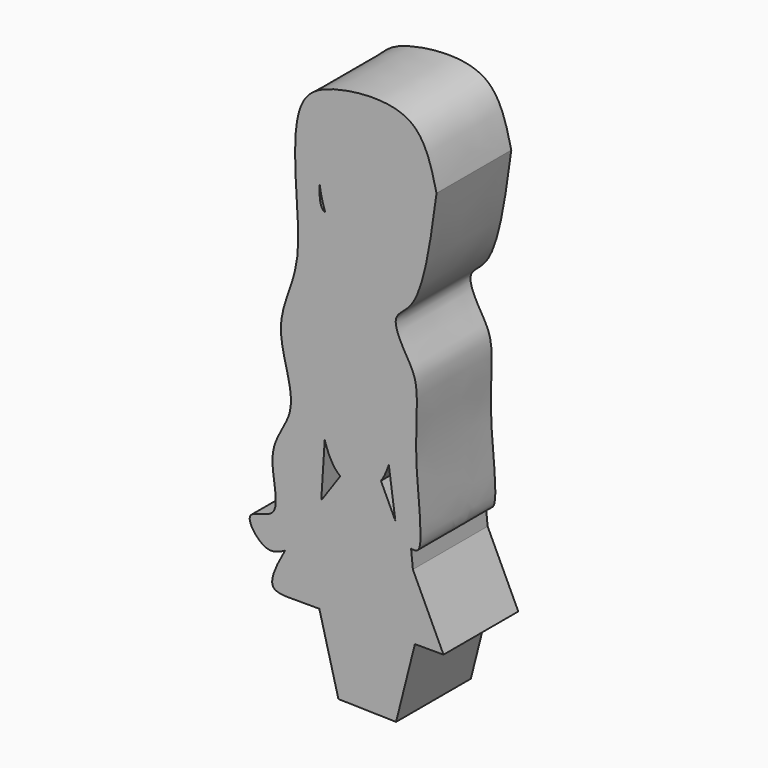
from build123d import *

# Parameters (mm, degrees)
F1_DEPTH = 25.4


with BuildPart() as f1:
    # F0 (on Front) → F1 (new body)
    with BuildSketch(Plane.XZ):
        with BuildLine():
            add(Edge.make_bspline(
                [(-13.2597442659, 48.0586274406), (-13.5977464023, 50.6112678955), (-13.8470723957, 57.8086655511), (-13.1131117441, 63.740427035), (-9.6694547683, 65.7902136445)],
                knots=[0.8065998572, 0.8065998572, 0.8065998572, 0.8065998572, 0.8751143357, 1, 1, 1, 1], degree=3))
            add(Edge.make_bspline(
                [(-9.6694547683, 65.7902136445), (-5.0770227001, 68.5237918796), (8.754968388, 67.9170672824), (13.1442032737, 62.5296557289), (13.9137207846, 60.7951997848)],
                knots=[0, 0, 0, 0, 0.1665464748, 0.23330744, 0.23330744, 0.23330744, 0.23330744], degree=3))
            add(Edge.make_bspline(
                [(13.9137207846, 60.7951997848), (14.5365060561, 59.3914713436), (15.6047629812, 54.0176064848), (14.0449258965, 45.1178162392), (7.561997369, 35.3712418653), (4.3727098317, 32.8274617106)],
                knots=[0.23330744, 0.23330744, 0.23330744, 0.23330744, 0.2873383688, 0.4230765743, 0.5331132448, 0.5331132448, 0.5331132448, 0.5331132448], degree=3))
            add(Edge.make_bspline(
                [(4.3727098317, 32.8274617106), (3.6723806459, 29.8240940225), (2.316637011, 24.0404033145), (4.425251651, 16.2436942218), (6.4598966618, 12.9076730343), (7.3942886665, 11.3758295774)],
                knots=[0, 0, 0, 0, 0.3683955853, 0.7100495981, 1, 1, 1, 1], degree=3))
            add(Edge.make_bspline(
                [(7.3942886665, 11.3758295774), (8.8184184197, -2.9290787173), (10.2432882502, -17.2336376752), (11.667567898, -31.5384752155)],
                knots=[0, 0, 0, 0, 43.1265648658, 43.1265648658, 43.1265648658, 43.1265648658], degree=3))
            add(Edge.make_bspline(
                [(18.5805205256, 55.7415634394), (16.9604621778, 43.7962208668), (14.5923827816, 26.3354173288), (5.783112798, 23.025573274), (9.9611159632, 14.6191299816), (14.2829401574, 8.3648794745), (11.7982647785, -8.4718891545), (15.6711855516, -32.1567528805), (12.4305942317, -31.6563107137), (11.667567898, -31.5384752155)],
                knots=[0, 0, 0, 0, 0.2296881978, 0.3357415022, 0.4503590021, 0.5643656145, 0.7444344835, 0.9398265709, 1, 1, 1, 1], degree=3))
            add(Edge.make_bspline(
                [(18.5805205256, 55.7415634394), (17.1329290258, 61.7846025086), (14.1281204981, 74.3283175814), (-8.5896728026, 72.8654786115), (-20.7194357662, 66.8136292861), (-19.5948869652, 43.7186228989), (-18.5533462423, 29.7113103857), (-20.7946125304, 20.6272816454), (-25.134054069, 10.2812154641), (-21.264747451, -1.7794824434), (-20.2945141104, -11.0677644833), (-28.6889299444, -20.5489013554), (-22.080213584, -37.1533798953), (-35.2491774446, -36.1367283315), (-28.1127555437, -45.9231665153), (-24.3435984622, -44.0537302743), (-22.6038616138, -43.1667872706)],
                knots=[0, 0, 0, 0, 0.085428964, 0.1772788288, 0.2494957552, 0.3459393214, 0.4258178937, 0.4882638252, 0.5568299207, 0.6301735859, 0.6919027853, 0.7637951512, 0.8404855359, 0.8945923927, 0.950900518, 1, 1, 1, 1], degree=3))
            add(Edge.make_bspline(
                [(-12.7485493713, -27.9239041306), (-16.6095460872, -33.5399624759), (-20.1444244224, -38.8530041581), (-22.6038616138, -43.1667872706)],
                knots=[0.1336483622, 0.1336483622, 0.1336483622, 0.1336483622, 0.4407324334, 0.4407324334, 0.4407324334, 0.4407324334], degree=3))
            add(Edge.make_bspline(
                [(-11.8084209481, -13.1750907084), (-12.1196551239, -18.0980314336), (-12.4373151954, -23.0009634054), (-12.7485493713, -27.9239041306)],
                knots=[0, 0, 0, 0, 14.7787461854, 14.7787461854, 14.7787461854, 14.7787461854], degree=3))
            add(Edge.make_bspline(
                [(-11.8084209481, -13.1750907084), (-13.8312312099, -6.5254381988), (-14.4995019899, 3.1835847003), (-15.1677727699, 12.8926075995)],
                knots=[0.7333685705, 0.7333685705, 0.7333685705, 0.7333685705, 1, 1, 1, 1], degree=3))
            add(Edge.make_bspline(
                [(-6.6413877679, 33.3635374314), (-6.2702296071, 30.7940506233), (-5.4996297901, 25.4655688344), (-8.9210699083, 16.2139387081), (-13.1930747657, 13.9425430583), (-15.1677727699, 12.8926075995)],
                knots=[0, 0, 0, 0, 0.3336593067, 0.6920012702, 1, 1, 1, 1], degree=3))
            add(Edge.make_bspline(
                [(-6.6413877679, 33.3635374314), (-8.1182076926, 34.7468870359), (-10.0297540913, 37.3896335016), (-11.3071284072, 40.3375022756), (-11.6578137626, 41.2990598225)],
                knots=[0.6602569137, 0.6602569137, 0.6602569137, 0.6602569137, 0.7180952928, 0.7451794293, 0.7451794293, 0.7451794293, 0.7451794293], degree=3))
            add(Edge.make_bspline(
                [(-11.6578137761, 41.2990598059), (-13.2743628001, 41.8800629418), (-13.2500921799, 44.9736955763), (-13.2597442659, 48.0586274406)],
                knots=[0.6826892363, 0.6826892363, 0.6826892363, 0.6826892363, 1, 1, 1, 1], degree=3))
        make_face()
        with BuildLine():
            add(Edge.make_bspline(
                [(-9.6694547683, 65.7902136445), (-5.0770227001, 68.5237918796), (8.754968388, 67.9170672824), (13.1442032737, 62.5296557289), (13.9137207846, 60.7951997848)],
                knots=[0, 0, 0, 0, 0.1665464748, 0.23330744, 0.23330744, 0.23330744, 0.23330744], degree=3))
            add(Edge.make_bspline(
                [(-13.2597442659, 48.0586274406), (-13.5977464023, 50.6112678955), (-13.8470723957, 57.8086655511), (-13.1131117441, 63.740427035), (-9.6694547683, 65.7902136445)],
                knots=[0.8065998572, 0.8065998572, 0.8065998572, 0.8065998572, 0.8751143357, 1, 1, 1, 1], degree=3))
            add(Edge.make_bspline(
                [(-11.6578137626, 41.2990598225), (-12.4530853654, 43.4796453527), (-12.9567391737, 45.7702896672), (-13.2597442659, 48.0586274406)],
                knots=[0.7451794293, 0.7451794293, 0.7451794293, 0.7451794293, 0.8065998572, 0.8065998572, 0.8065998572, 0.8065998572], degree=3))
            add(Edge.make_bspline(
                [(13.9137207846, 60.7951997848), (2.8933144958, 50.429697228), (-8.1798333223, 40.0490405239), (-11.6578137535, 41.2990597978)],
                knots=[0, 0, 0, 0, 0.6826892348, 0.6826892348, 0.6826892348, 0.6826892348], degree=3))
        make_face()
        with BuildLine():
            add(Edge.make_bspline(
                [(13.9137207846, 60.7951997848), (14.5365060561, 59.3914713436), (15.6047629812, 54.0176064848), (14.0449258965, 45.1178162392), (7.561997369, 35.3712418653), (4.3727098317, 32.8274617106)],
                knots=[0.23330744, 0.23330744, 0.23330744, 0.23330744, 0.2873383688, 0.4230765743, 0.5331132448, 0.5331132448, 0.5331132448, 0.5331132448], degree=3))
            add(Edge.make_bspline(
                [(13.9137207846, 60.7951997848), (2.8933144958, 50.429697228), (-8.1798333223, 40.0490405239), (-11.6578137535, 41.2990597978)],
                knots=[0, 0, 0, 0, 0.6826892348, 0.6826892348, 0.6826892348, 0.6826892348], degree=3))
            add(Edge.make_bspline(
                [(-6.6413877679, 33.3635374314), (-8.1182076926, 34.7468870359), (-10.0297540913, 37.3896335016), (-11.3071284072, 40.3375022756), (-11.6578137626, 41.2990598225)],
                knots=[0.6602569137, 0.6602569137, 0.6602569137, 0.6602569137, 0.7180952928, 0.7451794293, 0.7451794293, 0.7451794293, 0.7451794293], degree=3))
            add(Edge.make_bspline(
                [(4.3727098317, 32.8274617106), (2.9498352275, 31.6925749566), (-0.8831222645, 29.691479536), (-4.6484495647, 31.4967355087), (-6.6413877679, 33.3635374314)],
                knots=[0.5331132448, 0.5331132448, 0.5331132448, 0.5331132448, 0.5822052073, 0.6602569137, 0.6602569137, 0.6602569137, 0.6602569137], degree=3))
        make_face()
        with BuildLine():
            add(Edge.make_bspline(
                [(4.3727098317, 32.8274617106), (3.6723806459, 29.8240940225), (2.316637011, 24.0404033145), (4.425251651, 16.2436942218), (6.4598966618, 12.9076730343), (7.3942886665, 11.3758295774)],
                knots=[0, 0, 0, 0, 0.3683955853, 0.7100495981, 1, 1, 1, 1], degree=3))
            add(Edge.make_bspline(
                [(4.3727098317, 32.8274617106), (2.9498352275, 31.6925749566), (-0.8831222645, 29.691479536), (-4.6484495647, 31.4967355087), (-6.6413877679, 33.3635374314)],
                knots=[0.5331132448, 0.5331132448, 0.5331132448, 0.5331132448, 0.5822052073, 0.6602569137, 0.6602569137, 0.6602569137, 0.6602569137], degree=3))
            add(Edge.make_bspline(
                [(-6.6413877679, 33.3635374314), (-6.2702296071, 30.7940506233), (-5.4996297901, 25.4655688344), (-8.9210699083, 16.2139387081), (-13.1930747657, 13.9425430583), (-15.1677727699, 12.8926075995)],
                knots=[0, 0, 0, 0, 0.3336593067, 0.6920012702, 1, 1, 1, 1], degree=3))
            add(Edge.make_bspline(
                [(-15.1677727699, 12.8926075995), (-11.2202851493, 11.2914109173), (-3.5354144526, 8.17424105), (3.8180690975, 10.3282637453), (7.3942886665, 11.3758295774)],
                knots=[0, 0, 0, 0, 0.5136700117, 1, 1, 1, 1], degree=3))
        make_face()
        with BuildLine():
            add(Edge.make_bspline(
                [(7.3942886665, 11.3758295774), (7.4809183559, 2.1480170491), (7.5675480452, -7.0797954793), (5.6052811607, -13.4339725009)],
                knots=[0, 0, 0, 0, 0.2824189835, 0.2824189835, 0.2824189835, 0.2824189835], degree=3))
            add(Edge.make_bspline(
                [(-15.1677727699, 12.8926075995), (-11.2202851493, 11.2914109173), (-3.5354144526, 8.17424105), (3.8180690975, 10.3282637453), (7.3942886665, 11.3758295774)],
                knots=[0, 0, 0, 0, 0.5136700117, 1, 1, 1, 1], degree=3))
            add(Edge.make_bspline(
                [(-11.8084209481, -13.1750907084), (-13.8312312099, -6.5254381988), (-14.4995019899, 3.1835847003), (-15.1677727699, 12.8926075995)],
                knots=[0.7333685705, 0.7333685705, 0.7333685705, 0.7333685705, 1, 1, 1, 1], degree=3))
            add(Edge.make_bspline(
                [(-7.583886385, -20.4764921218), (-9.4445070613, -19.0645807661), (-10.7960911687, -16.5029565912), (-11.8084209481, -13.1750907084)],
                knots=[0.5999309757, 0.5999309757, 0.5999309757, 0.5999309757, 0.7333685705, 0.7333685705, 0.7333685705, 0.7333685705], degree=3))
            add(Edge.make_bspline(
                [(3.4724624485, -17.9735615732), (3.272980363, -18.2531337634), (0.3808615018, -21.924396042), (-4.4840378333, -22.8287778009), (-7.583886385, -20.4764921218)],
                knots=[0.3602725637, 0.3602725637, 0.3602725637, 0.3602725637, 0.3776200337, 0.5999309757, 0.5999309757, 0.5999309757, 0.5999309757], degree=3))
            add(Edge.make_bspline(
                [(5.6052811607, -13.4339725009), (5.0643490302, -15.185609111), (4.3677166016, -16.7188716407), (3.4724624485, -17.9735615732)],
                knots=[0.2824189835, 0.2824189835, 0.2824189835, 0.2824189835, 0.3602725637, 0.3602725637, 0.3602725637, 0.3602725637], degree=3))
        make_face()
        with BuildLine():
            add(Edge.make_bspline(
                [(7.3942886665, 11.3758295774), (8.8184184197, -2.9290787173), (10.2432882502, -17.2336376752), (11.667567898, -31.5384752155)],
                knots=[0, 0, 0, 0, 43.1265648658, 43.1265648658, 43.1265648658, 43.1265648658], degree=3))
            add(Edge.make_bspline(
                [(7.3942886665, 11.3758295774), (7.4809183559, 2.1480170491), (7.5675480452, -7.0797954793), (5.6052811607, -13.4339725009)],
                knots=[0, 0, 0, 0, 0.2824189835, 0.2824189835, 0.2824189835, 0.2824189835], degree=3))
            add(Edge.make_bspline(
                [(7.3942886665, -26.2981797794), (6.7973669435, -22.0099297555), (6.2022028837, -17.7222225248), (5.6052811607, -13.4339725009)],
                knots=[0, 0, 0, 0, 12.9880089606, 12.9880089606, 12.9880089606, 12.9880089606], degree=3))
            add(Edge.make_bspline(
                [(12.149010106, -36.3741251388), (10.5633985271, -33.0149740546), (8.9776998193, -29.6557608018), (7.3942886665, -26.2981797794)],
                knots=[19.5261849929, 19.5261849929, 19.5261849929, 19.5261849929, 30.6617591048, 30.6617591048, 30.6617591048, 30.6617591048], degree=3))
            add(Edge.make_bspline(
                [(11.667567898, -31.5384752155), (11.8280567619, -33.1503546867), (11.9885381323, -34.762237695), (12.149010106, -36.3741251388)],
                knots=[43.1265648658, 43.1265648658, 43.1265648658, 43.1265648658, 47.9860974801, 47.9860974801, 47.9860974801, 47.9860974801], degree=3))
        make_face()
        with BuildLine():
            add(Edge.make_bspline(
                [(7.3942886665, -26.2981797794), (6.0850016835, -23.5218717311), (4.777278762, -20.7466796816), (3.4724624485, -17.9735615732)],
                knots=[30.6617591048, 30.6617591048, 30.6617591048, 30.6617591048, 39.8695142787, 39.8695142787, 39.8695142787, 39.8695142787], degree=3))
            add(Edge.make_bspline(
                [(3.4724624485, -17.9735615732), (3.272980363, -18.2531337634), (0.3808615018, -21.924396042), (-4.4840378333, -22.8287778009), (-7.583886385, -20.4764921218)],
                knots=[0.3602725637, 0.3602725637, 0.3602725637, 0.3602725637, 0.3776200337, 0.5999309757, 0.5999309757, 0.5999309757, 0.5999309757], degree=3))
            add(Edge.make_bspline(
                [(-7.583886385, -20.4764921218), (-9.3260312058, -22.9780946851), (-11.0681760267, -25.4796972484), (-12.7485493713, -27.9239041306)],
                knots=[0, 0, 0, 0, 0.1336483622, 0.1336483622, 0.1336483622, 0.1336483622], degree=3))
            add(Edge.make_bspline(
                [(-12.7485493713, -27.9239041306), (-16.6095460872, -33.5399624759), (-20.1444244224, -38.8530041581), (-22.6038616138, -43.1667872706)],
                knots=[0.1336483622, 0.1336483622, 0.1336483622, 0.1336483622, 0.4407324334, 0.4407324334, 0.4407324334, 0.4407324334], degree=3))
            add(Edge.make_bspline(
                [(-22.6038616138, -43.1667872706), (-25.1173571376, -47.5753871658), (-27.5948677622, -53.5718639736), (-23.9652974865, -53.8938759719), (-22.3724655807, -54.0351904929)],
                knots=[0.4407324334, 0.4407324334, 0.4407324334, 0.4407324334, 0.7545662003, 1, 1, 1, 1], degree=3))
            add(Edge.make_bspline(
                [(-22.3724655807, -54.0351904929), (-19.3389107784, -54.0351904929), (-16.305355976, -54.0351904929), (-13.2718011737, -54.0351904929)],
                knots=[0, 0, 0, 0, 9.100664407, 9.100664407, 9.100664407, 9.100664407], degree=3))
            add(Edge.make_bspline(
                [(-13.2718011737, -54.0351904929), (-8.8478674491, -54.0351904929), (-4.4239337246, -54.0351904929), (0, -54.0351904929)],
                knots=[9.100664407, 9.100664407, 9.100664407, 9.100664407, 22.3724655807, 22.3724655807, 22.3724655807, 22.3724655807], degree=3))
            add(Edge.make_bspline(
                [(0, -54.0351904929), (4.2343363166, -54.0351904929), (8.4686726332, -54.0351904929), (12.7030089498, -54.0351904929)],
                knots=[22.3724655807, 22.3724655807, 22.3724655807, 22.3724655807, 35.0754745305, 35.0754745305, 35.0754745305, 35.0754745305], degree=3))
            add(Edge.make_bspline(
                [(12.7030089498, -54.0351904929), (15.294170628, -54.0351904929), (17.8853323062, -54.0351904929), (20.4764939845, -54.0351904929)],
                knots=[35.0754745305, 35.0754745305, 35.0754745305, 35.0754745305, 42.8489595652, 42.8489595652, 42.8489595652, 42.8489595652], degree=3))
            add(Edge.make_bspline(
                [(20.4764939845, -54.0351904929), (17.7094694232, -48.1544501636), (14.9293737143, -42.2643832278), (12.149010106, -36.3741251388)],
                knots=[0, 0, 0, 0, 19.5261849929, 19.5261849929, 19.5261849929, 19.5261849929], degree=3))
            add(Edge.make_bspline(
                [(12.149010106, -36.3741251388), (10.5633985271, -33.0149740546), (8.9776998193, -29.6557608018), (7.3942886665, -26.2981797794)],
                knots=[19.5261849929, 19.5261849929, 19.5261849929, 19.5261849929, 30.6617591048, 30.6617591048, 30.6617591048, 30.6617591048], degree=3))
        make_face()
        with BuildLine():
            add(Edge.make_bspline(
                [(12.7030089498, -54.0351904929), (10.9966344511, -60.7974901795), (9.2902599523, -67.5597898662), (7.5838854536, -74.3220895529)],
                knots=[0, 0, 0, 0, 20.9228033217, 20.9228033217, 20.9228033217, 20.9228033217], degree=3))
            add(Edge.make_bspline(
                [(0, -54.0351904929), (4.2343363166, -54.0351904929), (8.4686726332, -54.0351904929), (12.7030089498, -54.0351904929)],
                knots=[22.3724655807, 22.3724655807, 22.3724655807, 22.3724655807, 35.0754745305, 35.0754745305, 35.0754745305, 35.0754745305], degree=3))
            add(Edge.make_bspline(
                [(0, -54.0351904929), (0, -60.7363293296), (0, -67.4374681664), (0, -74.1386070032)],
                knots=[0, 0, 0, 0, 20.1034165103, 20.1034165103, 20.1034165103, 20.1034165103], degree=3))
            add(Edge.make_bspline(
                [(0, -74.1386070032), (2.5279618179, -74.1997678531), (5.0559236358, -74.260928703), (7.5838854536, -74.3220895529)],
                knots=[8.0918462485, 8.0918462485, 8.0918462485, 8.0918462485, 15.6779509419, 15.6779509419, 15.6779509419, 15.6779509419], degree=3))
        make_face()
        with BuildLine():
            add(Edge.make_bspline(
                [(0, -54.0351904929), (0, -60.7363293296), (0, -67.4374681664), (0, -74.1386070032)],
                knots=[0, 0, 0, 0, 20.1034165103, 20.1034165103, 20.1034165103, 20.1034165103], degree=3))
            add(Edge.make_bspline(
                [(-13.2718011737, -54.0351904929), (-8.8478674491, -54.0351904929), (-4.4239337246, -54.0351904929), (0, -54.0351904929)],
                knots=[9.100664407, 9.100664407, 9.100664407, 9.100664407, 22.3724655807, 22.3724655807, 22.3724655807, 22.3724655807], degree=3))
            add(Edge.make_bspline(
                [(-13.2718011737, -54.0351904929), (-11.5443604688, -60.6710910797), (-9.8169197639, -67.3069916666), (-8.089479059, -73.9428922534)],
                knots=[0, 0, 0, 0, 20.5711704063, 20.5711704063, 20.5711704063, 20.5711704063], degree=3))
            add(Edge.make_bspline(
                [(-8.089479059, -73.9428922534), (-5.3929860393, -74.0081305033), (-2.6964930197, -74.0733687532), (0, -74.1386070032)],
                knots=[0, 0, 0, 0, 8.0918462485, 8.0918462485, 8.0918462485, 8.0918462485], degree=3))
        make_face()
    extrude(amount=F1_DEPTH)


solid = f1.part
